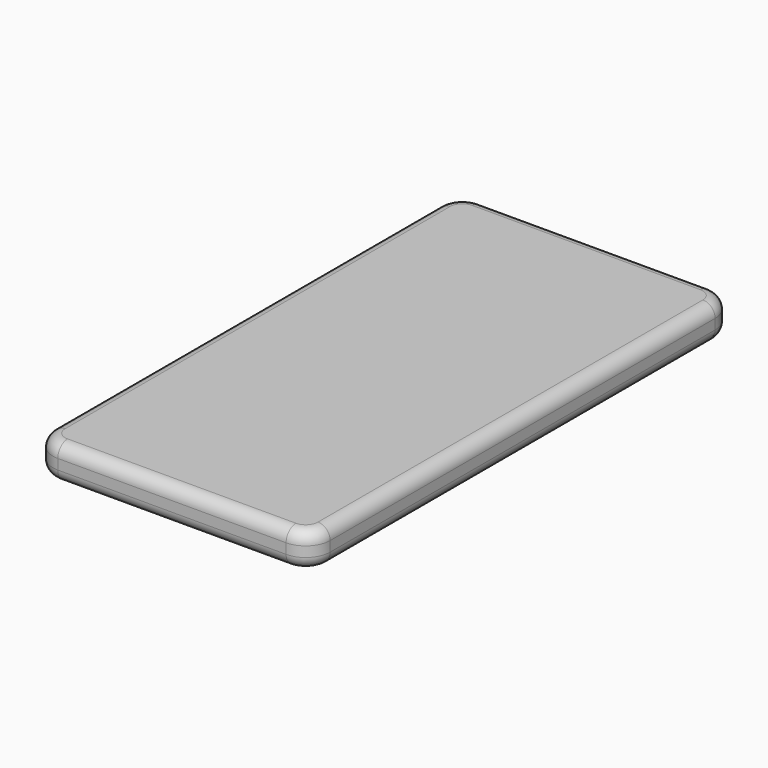
from build123d import *

# Parameters (mm, degrees)
F0_W         = 68
F0_H         = 130
F1_DEPTH     = 8.5
F2_R         = 3
F3_T1_DEPTH  = 8.5
F3_T4_ANGLE  = 90
F3_T6_ANGLE  = 90
F3_T8_ANGLE  = 90
F3_T10_ANGLE = 90
F3_T12_ANGLE = 90
F3_T14_ANGLE = 90
F3_T16_ANGLE = 90
F3_T18_ANGLE = 90


# Not quite as in the source:
# - a fillet or chamfer that OpenCascade refuses, or shapes differently, is made with other operations: its cross-section is extruded or revolved along the edge and cut away or added


with BuildPart() as f1:
    # F0 (on Top) → F1 (new body)
    with BuildSketch(Plane.XY):
        with Locations((34, 65)):
            Rectangle(F0_W, F0_H)
    extrude(amount=F1_DEPTH)

    # F2
    f2_edges = [f1.edges().sort_by_distance(p)[0] for p in [
        (0, 65, 8.5),
        (0, 65, 0),
        (68, 65, 8.5),
        (68, 65, 0),
        (34, 0, 0),
        (34, 0, 8.5),
        (34, 130, 8.5),
        (34, 130, 0),
    ]]
    fillet(f2_edges, radius=F2_R)

    # F3: fillet of radius 6 on 4 edges, made by hand

    # F3_s2 → F3_t1 (cut)
    with BuildSketch(Plane.XY):
        with BuildLine():
            ThreePointArc((0, 6), (1.7573593129, 1.7573593129), (6, 0))
            Line((6, 0), (0, 0))
            Line((0, 0), (0, 6))
        make_face()
        with BuildLine():
            ThreePointArc((62, 0), (66.2426406871, 1.7573593129), (68, 6))
            Line((68, 6), (68, 0))
            Line((68, 0), (62, 0))
        make_face()
        with BuildLine():
            ThreePointArc((62, 130), (66.2426406871, 128.2426406871), (68, 124))
            Line((68, 124), (68, 130))
            Line((68, 130), (62, 130))
        make_face()
        with BuildLine():
            ThreePointArc((0, 124), (1.7573593129, 128.2426406871), (6, 130))
            Line((6, 130), (0, 130))
            Line((0, 130), (0, 124))
        make_face()
    extrude(amount=F3_T1_DEPTH, mode=Mode.SUBTRACT)

    # F3_s3 → F3_t4 (revolve, cut)
    with BuildSketch(Plane.XZ.offset(-124)):
        with BuildLine():
            ThreePointArc((3, 0), (0.8786796564, 0.8786796564), (0, 3))
            Line((0, 3), (0, 0))
            Line((0, 0), (3, 0))
        make_face()
    revolve(axis=Axis((6, 124, 0), (0, 0, -1)), revolution_arc=F3_T4_ANGLE, mode=Mode.SUBTRACT)

    # F3_s5 → F3_t6 (revolve, cut)
    with BuildSketch(Plane.YZ.offset(6)):
        with BuildLine():
            ThreePointArc((127, 8.5), (129.1213203436, 7.6213203436), (130, 5.5))
            Line((130, 5.5), (130, 8.5))
            Line((130, 8.5), (127, 8.5))
        make_face()
    revolve(axis=Axis((6, 124, 8.5), (0, 0, 1)), revolution_arc=F3_T6_ANGLE, mode=Mode.SUBTRACT)

    # F3_s7 → F3_t8 (revolve, cut)
    with BuildSketch(Plane.YZ.offset(62)):
        with BuildLine():
            ThreePointArc((127, 0), (129.1213203436, 0.8786796564), (130, 3))
            Line((130, 3), (130, 0))
            Line((130, 0), (127, 0))
        make_face()
    revolve(axis=Axis((62, 124, 0), (0, 0, -1)), revolution_arc=F3_T8_ANGLE, mode=Mode.SUBTRACT)

    # F3_s9 → F3_t10 (revolve, cut)
    with BuildSketch(Plane.XZ.offset(-124)):
        with BuildLine():
            ThreePointArc((65, 8.5), (67.1213203436, 7.6213203436), (68, 5.5))
            Line((68, 5.5), (68, 8.5))
            Line((68, 8.5), (65, 8.5))
        make_face()
    revolve(axis=Axis((62, 124, 8.5), (0, 0, 1)), revolution_arc=F3_T10_ANGLE, mode=Mode.SUBTRACT)

    # F3_s11 → F3_t12 (revolve, cut)
    with BuildSketch(Plane.XZ.offset(-6)):
        with BuildLine():
            ThreePointArc((65, 0), (67.1213203436, 0.8786796564), (68, 3))
            Line((68, 3), (68, 0))
            Line((68, 0), (65, 0))
        make_face()
    revolve(axis=Axis((62, 6, 0), (0, 0, -1)), revolution_arc=F3_T12_ANGLE, mode=Mode.SUBTRACT)

    # F3_s13 → F3_t14 (revolve, cut)
    with BuildSketch(Plane.YZ.offset(62)):
        with BuildLine():
            ThreePointArc((3, 8.5), (0.8786796564, 7.6213203436), (0, 5.5))
            Line((0, 5.5), (0, 8.5))
            Line((0, 8.5), (3, 8.5))
        make_face()
    revolve(axis=Axis((62, 6, 8.5), (0, 0, 1)), revolution_arc=F3_T14_ANGLE, mode=Mode.SUBTRACT)

    # F3_s15 → F3_t16 (revolve, cut)
    with BuildSketch(Plane.YZ.offset(6)):
        with BuildLine():
            ThreePointArc((3, 0), (0.8786796564, 0.8786796564), (0, 3))
            Line((0, 3), (0, 0))
            Line((0, 0), (3, 0))
        make_face()
    revolve(axis=Axis((6, 6, 0), (0, 0, -1)), revolution_arc=F3_T16_ANGLE, mode=Mode.SUBTRACT)

    # F3_s17 → F3_t18 (revolve, cut)
    with BuildSketch(Plane.XZ.offset(-6)):
        with BuildLine():
            ThreePointArc((3, 8.5), (0.8786796564, 7.6213203436), (0, 5.5))
            Line((0, 5.5), (0, 8.5))
            Line((0, 8.5), (3, 8.5))
        make_face()
    revolve(axis=Axis((6, 6, 8.5), (0, 0, 1)), revolution_arc=F3_T18_ANGLE, mode=Mode.SUBTRACT)


solid = f1.part
